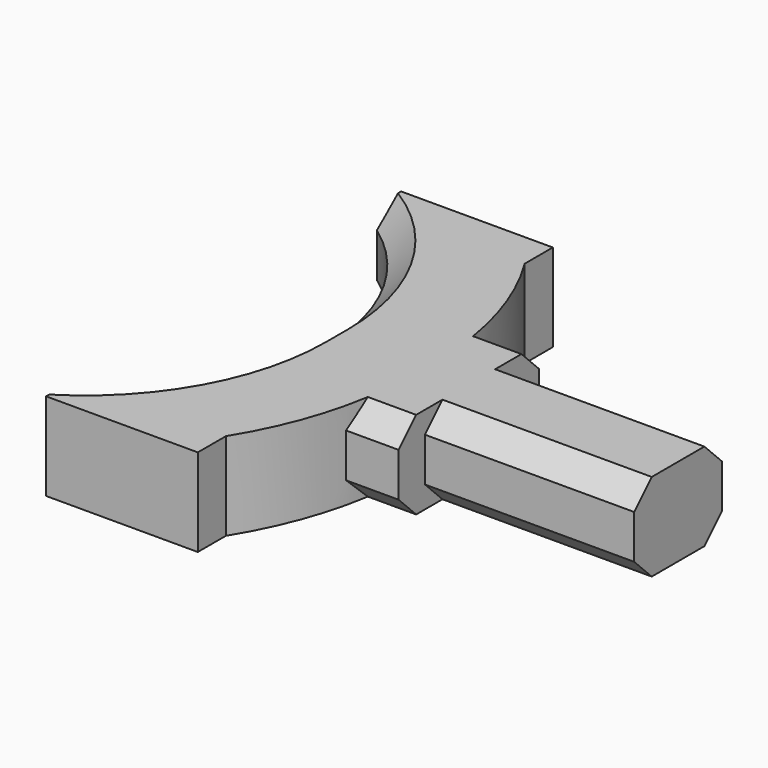
from build123d import *

# Parameters (mm, degrees)
F1_DEPTH = 2
F2_SIZE  = 1


with BuildPart() as f1:
    # F0 (on Top) → F1 (new body, symmetric)
    with BuildSketch(Plane.XY):
        with BuildLine():
            Line((-64.3336782856, 36.2610286334), (-64.3336782856, 34.8834841531))
            Line((-64.3336782856, 34.8834841531), (-57.4157565349, 34.8834841531))
            Line((-57.4157565349, 34.8834841531), (-57.4157565349, 36.4834841531))
            ThreePointArc((-57.4157565349, 36.4834841531), (-56.2994751301, 38.665413461), (-55.5534152324, 41))
            Line((-55.5534152324, 41), (-53.1534152324, 41))
            Line((-53.1534152324, 41), (-53.1534152324, 42.5))
            Line((-53.1534152324, 42.5), (-43.6123318144, 42.5))
            Line((-43.6123318144, 42.5), (-43.6123318144, 45))
            Line((-43.6123318144, 45), (-43.6123318144, 47.5))
            Line((-43.6123318144, 47.5), (-53.1534152324, 47.5))
            Line((-53.1534152324, 47.5), (-53.1534152324, 49))
            Line((-53.1534152324, 49), (-55.5534152324, 49))
            ThreePointArc((-55.5534152324, 49), (-56.2994751301, 51.334586539), (-57.4157565349, 53.5165158469))
            Line((-57.4157565349, 53.5165158469), (-57.4157565349, 55.1165158469))
            Line((-57.4157565349, 55.1165158469), (-64.3336782856, 55.1165158469))
            Line((-64.3336782856, 55.1165158469), (-64.3336782856, 53.7389713666))
            ThreePointArc((-64.3336782856, 53.7389713666), (-61.2693193587, 50.1809672734), (-60.1668349206, 45.6165158469))
            Line((-60.1668349206, 45.6165158469), (-60.1668349206, 44.3834841531))
            ThreePointArc((-60.1668349206, 44.3834841531), (-61.2693193587, 39.8190327266), (-64.3336782856, 36.2610286334))
        make_face()
    extrude(amount=F1_DEPTH, both=True)

    # F2
    f2_edges = [f1.edges().sort_by_distance(p)[0] for p in [
        (-54.353415, 49, -2),
        (-54.353415, 49, 2),
        (-54.353415, 41, 2),
        (-54.353415, 41, -2),
        (-48.382874, 47.5, -2),
        (-48.382874, 42.5, -2),
        (-48.382874, 47.5, 2),
        (-48.382874, 42.5, 2),
        (-61.269319, 50.180967, 2),
        (-61.269319, 39.819033, -2),
        (-61.269319, 39.819033, 2),
        (-60.166835, 45, -2),
        (-60.166835, 45, 2),
        (-61.269319, 50.180967, -2),
    ]]
    chamfer(f2_edges, length=F2_SIZE)


solid = f1.part
